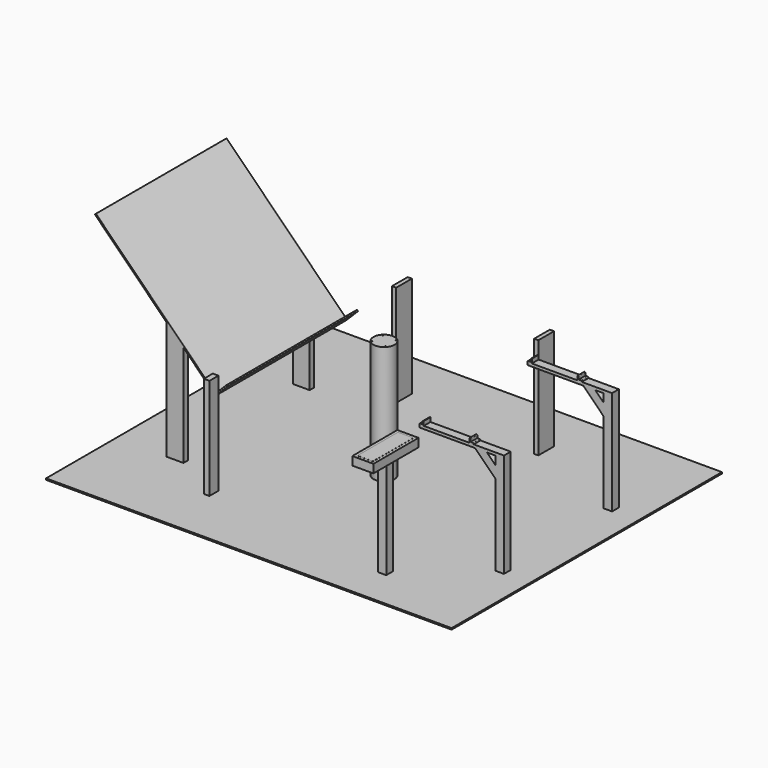
from build123d import *

# Parameters (mm, degrees)
F0_W          = 3657.6
F0_H          = 3048
F1_DEPTH      = 12.7
F2_R          = 95.25
F2_R_2        = 4.25
F3_DEPTH      = 1066.8
F4_W          = 38.1
F4_H          = 177.8
F4_W_2        = 50.8
F4_H_2        = 101.6
F4_W_3        = 76.2
F4_H_3        = 76.2
F5_DEPTH      = 914.4
F6_W          = 152.4
F6_H          = 50.8
F7_DEPTH      = 914.4
F9_DEPTH      = 736.6
F9_DEPTH_BACK = 736.6
F11_DEPTH     = 76.2
F13_DEPTH     = 76.2
F14_R         = 6.35
F15_W         = 190.5
F15_H         = 508
F16_DEPTH     = 76.2
F17_W         = 139.7
F17_H         = 457.2
F18_DEPTH     = 0.635


with BuildPart() as f1:
    # F0 (on Top) → F1 (new body)
    with BuildSketch(Plane.XY):
        Rectangle(F0_W, F0_H)
    extrude(amount=F1_DEPTH)

    # F2 (on face) → F3 (join)
    with BuildSketch(Plane.XY.offset(12.7)):
        Circle(F2_R)
        with Locations((-60.1040764009, -60.1040764009)):
            Circle(F2_R_2, mode=Mode.SUBTRACT)
        with Locations((60.1040764009, -60.1040764009)):
            Circle(F2_R_2, mode=Mode.SUBTRACT)
        with Locations((-60.1040764009, 60.1040764009)):
            Circle(F2_R_2, mode=Mode.SUBTRACT)
        with Locations((60.1040764009, 60.1040764009)):
            Circle(F2_R_2, mode=Mode.SUBTRACT)
    extrude(amount=F3_DEPTH)

    # F4 (on face) → F5 (join)
    with BuildSketch(Plane.XY.offset(12.7)):
        with Locations((-641.35, 1003.3)):
            Rectangle(F4_W, F4_H)
        with Locations((641.35, 1003.3)):
            Rectangle(F4_W, F4_H)
        with Locations((-787.4, -965.2)):
            Rectangle(F4_W_2, F4_H_2)
        with Locations((787.4, -965.2)):
            Rectangle(F4_W_2, F4_H_2)
        with Locations((1562.1, 609.6)):
            Rectangle(F4_W_3, F4_H_3)
        with Locations((1562.1, -609.6)):
            Rectangle(F4_W_3, F4_H_3)
        with Locations((927.1, -1143)):
            Rectangle(F4_W_3, F4_H_3)
    extrude(amount=F5_DEPTH)

    # F6 (on face) → F7 (join)
    with BuildSketch(Plane.XY.offset(12.7)):
        with Locations((-1295.4, 711.2)):
            Rectangle(F6_W, F6_H)
        with Locations((-1295.4, -711.2)):
            Rectangle(F6_W, F6_H)
    extrude(amount=F7_DEPTH)

    # F8 (on Front) → F9 (join, two sides)
    with BuildSketch(Plane.XZ) as f9_sk:
        Polygon((-1371.6, 1079.5), (-1371.6, 927.1), (-1219.2, 927.1), (-931.5674500676, 639.4674500676), (-823.8043766148, 747.2305235204), (-832.7846327359, 756.2107796415), (-931.5674500676, 657.4279623097), (-2009.1981845959, 1735.058696838), (-2018.178440717, 1726.078440717), align=None)
    extrude(amount=F9_DEPTH)
    extrude(f9_sk.sketch, amount=-F9_DEPTH_BACK)

    # F10 (on face) → F11 (join, through all)
    with BuildSketch(Plane.XZ.offset(647.7)):
        Polygon((1447.8, 927.1), (1600.2, 927.1), (1600.2, 952.5), (1327.15, 952.5), (1327.15, 962.025), (1298.575, 962.025), (1298.575, 990.6), (1289.05, 990.6), (1289.05, 952.5), (876.3, 952.5), (876.3, 990.6), (866.775, 990.6), (866.775, 962.025), (838.2, 962.025), (838.2, 927.1), (1340.0369265472, 927.1), (1524, 743.1369265472), (1524, 850.9), align=None)
    extrude(amount=-F11_DEPTH)

    # F12 (on face) → F13 (join, through all)
    with BuildSketch(Plane.XZ.offset(-571.5)):
        Polygon((1447.8, 927.1), (1600.2, 927.1), (1600.2, 952.5), (1327.15, 952.5), (1327.15, 962.025), (1298.575, 962.025), (1298.575, 990.6), (1289.05, 990.6), (1289.05, 952.5), (876.3, 952.5), (876.3, 990.6), (866.775, 990.6), (866.775, 962.025), (838.2, 962.025), (838.2, 927.1), (1340.0369265472, 927.1), (1600.2, 666.9369265472), (1600.2, 774.7), align=None)
    extrude(amount=-F13_DEPTH)

    # F14
    f14_edges = [f1.edges().sort_by_distance(p)[0] for p in [
        (866.775, -609.6, 990.6),
        (1298.575, -609.6, 990.6),
        (1327.15, -609.6, 962.025),
        (866.775, 609.6, 990.6),
        (838.2, 609.6, 962.025),
        (1298.575, 609.6, 990.6),
        (1327.15, 609.6, 962.025),
        (866.775, -609.6, 962.025),
        (838.2, -609.6, 962.025),
    ]]
    fillet(f14_edges, radius=F14_R)

    # F15 (on face) → F16 (join)
    with BuildSketch(Plane.XY.offset(927.1)):
        with Locations((927.1, -1143)):
            Rectangle(F15_W, F15_H)
    extrude(amount=F16_DEPTH)


with BuildPart() as f18:
    # F17 (on face) → F18 (new body)
    with BuildSketch(Plane.XY.offset(1003.3)):
        with Locations((927.1, -1143)):
            Rectangle(F17_W, F17_H)
    extrude(amount=F18_DEPTH)


solid = Compound([f1.part, f18.part])
